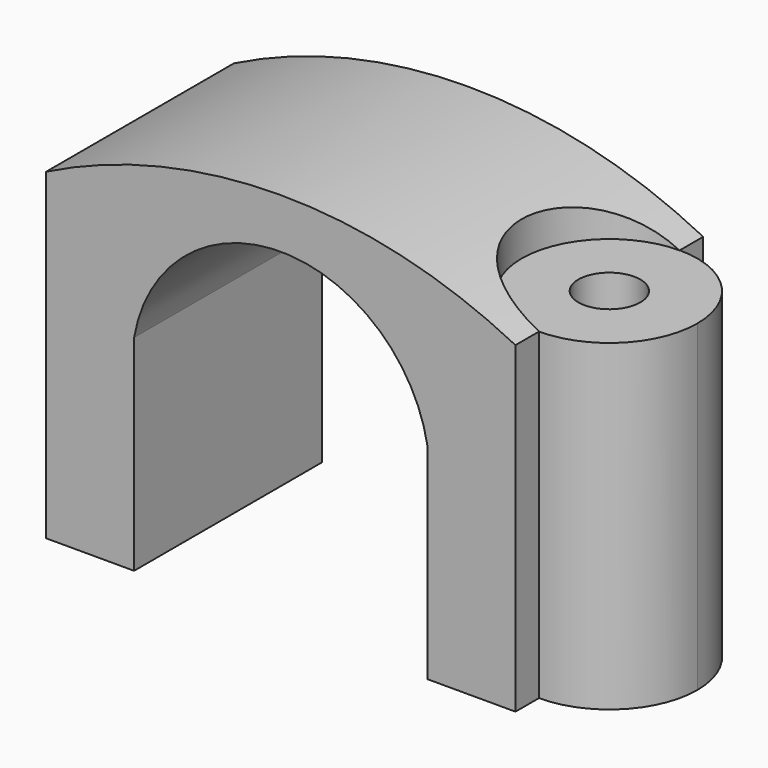
from build123d import *

# Parameters (mm, degrees)
F0_W      = 16
F0_H      = 8
F1_DEPTH  = 11
F3_DEPTH  = 11
F5_DEPTH  = 8
F6_W      = 10
F6_H      = 7
F7_DEPTH  = 25.4
F9_DEPTH  = 25.4
F10_R     = 2.9921817394
F11_DEPTH = 25.4
F12_R     = 1.0573915373
F13_DEPTH = 25.4


with BuildPart() as f1:
    # F0 (on Top) → F1 (new body)
    with BuildSketch(Plane.XY):
        with Locations((8, 4)):
            Rectangle(F0_W, F0_H)
    extrude(amount=F1_DEPTH)

    # F2 (on face) → F3 (join)
    with BuildSketch(Plane.XY.offset(11)):
        with BuildLine():
            Line((16, 7), (16, 1))
            ThreePointArc((16, 1), (18.1213203436, 1.8786796564), (19, 4))
            ThreePointArc((19, 4), (18.1213203436, 6.1213203436), (16, 7))
        make_face()
    extrude(amount=-F3_DEPTH)

    # F4 (on face) → F5 (join)
    with BuildSketch(Plane(origin=(0, 8, 0), x_dir=(-1, 0, 0), z_dir=(0, 1, 0))):
        with BuildLine():
            Line((-16, 11), (0, 11))
            ThreePointArc((0, 11), (-8, 12.9014484288), (-16, 11))
        make_face()
    extrude(amount=-F5_DEPTH)

    # F6 (on face) → F7 (cut)
    with BuildSketch(Plane(origin=(0, 8, 0), x_dir=(-1, 0, 0), z_dir=(0, 1, 0))):
        with Locations((-8, 3.5)):
            Rectangle(F6_W, F6_H)
    extrude(amount=-F7_DEPTH, mode=Mode.SUBTRACT)

    # F8 (on face) → F9 (cut)
    with BuildSketch(Plane(origin=(0, 8, 0), x_dir=(-1, 0, 0), z_dir=(0, 1, 0))):
        with BuildLine():
            Line((-13, 7), (-3, 7))
            ThreePointArc((-3, 7), (-8, 11.2036427481), (-13, 7))
        make_face()
    extrude(amount=-F9_DEPTH, mode=Mode.SUBTRACT)

    # F10 (on face) → F11 (cut)
    with BuildSketch(Plane.XY.offset(11)):
        with Locations((16, 4)):
            Circle(F10_R)
    extrude(amount=F11_DEPTH, mode=Mode.SUBTRACT)

    # F12 (on face) → F13 (cut)
    with BuildSketch(Plane.XY.offset(11)):
        with Locations((16, 4)):
            Circle(F12_R)
    extrude(amount=-F13_DEPTH, mode=Mode.SUBTRACT)


solid = f1.part
